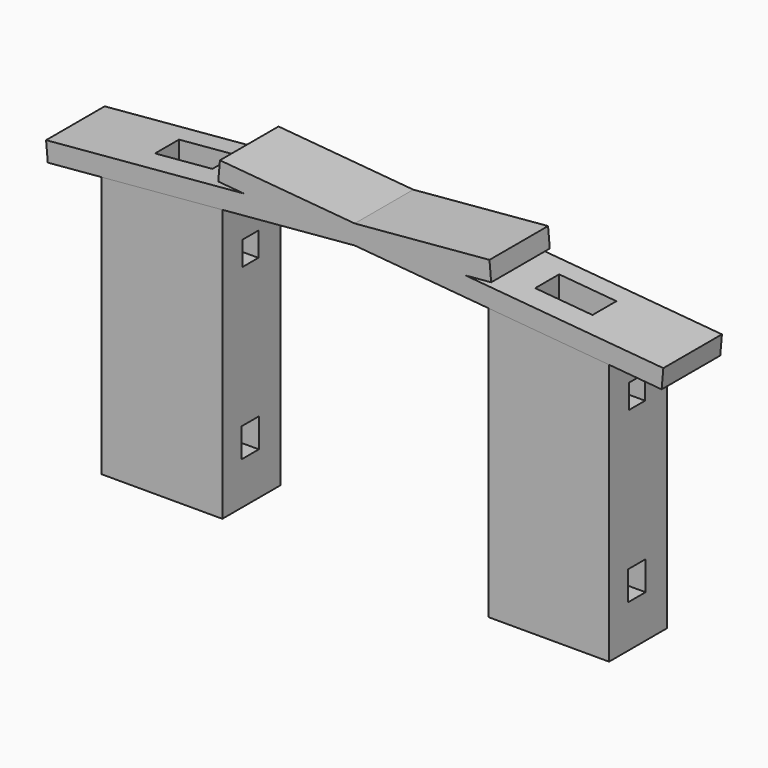
from build123d import *

# Parameters (mm, degrees)
F0_W      = 6.35
F0_H      = 6.35
F1_DEPTH  = 76.2
F3_W      = 78.9158530533
F3_H      = 6.5545327961
F4_DEPTH  = 5.08
F5_DEPTH  = 38.1
F7_DEPTH  = 25.4
F8_DEPTH  = 25.4
F9_DEPTH  = 12.7
F10_DEPTH = 12.7
F11_W     = 15.0663554668
F11_H     = 7.8755952418
F12_DEPTH = 88.9
F13_W     = 5.7417834178
F13_H     = 7.6454
F14_DEPTH = 2540
F15_W     = 5.208699964
F15_H     = 6.3248500228
F16_DEPTH = 25400


# Not quite as in the source:
# - a feature names something its author has since deleted; it is built from what else it names


with BuildPart() as f1:
    # F0 (on Top) → F1 (new body)
    with BuildSketch(Plane.XY):
        with Locations((-38.1329911691, -3.175)):
            Rectangle(F0_W, F0_H)
    extrude(amount=F1_DEPTH)

    # F3 (on face) → F4 (join)
    with BuildSketch(Plane(origin=(-6.9297761713, 0, 79.2077040846), x_dir=(0.9961946981, 0, 0.0871557427), z_dir=(0.0871557427, 0, -0.9961946981))):
        with Locations((3.0671004206, 3.2772663981)):
            Rectangle(F3_W, F3_H)
    extrude(amount=F4_DEPTH)

    # F5 (add): a face of the model
    f5_faces = [f1.faces().sort_by_distance(p)[0] for p in [
        (-42.9607486108, -3.2772663981, 73.5057000729),
    ]]
    extrude(f5_faces, amount=F5_DEPTH)

    # F6: F1 across plane


with BuildPart() as f1_1:
    add(f1.part)
    add(f1.part.mirror(Plane.YZ))

    # F7 (add): a face of the model
    f7_faces = [f1_1.faces().sort_by_distance(p)[0] for p in [
        (-41.3079911691, -3.175, 35.5502976126),
    ]]
    extrude(f7_faces, amount=F7_DEPTH)

    # F8 (add): a face of the model
    f8_faces = [f1_1.faces().sort_by_distance(p)[0] for p in [
        (41.3079911691, -3.175, 35.5502976126),
    ]]
    extrude(f8_faces, amount=F8_DEPTH)

    # F9 (add): a face of the model
    f9_faces = [f1_1.faces().sort_by_distance(p)[0] for p in [
        (0, -6.5545327961, 75.0015171841),
    ]]
    extrude(f9_faces, amount=F9_DEPTH)

    # F10 (add): faces of the model
    f10_faces = [f1_1.faces().sort_by_distance(p)[0] for p in [
        (-50.72839761, -6.35, 35.1382082279),
        (50.72839761, -6.35, 35.1382082279),
    ]]
    extrude(f10_faces, amount=F10_DEPTH)

    # F11 (on face) → F12 (cut)
    with BuildSketch(Plane(origin=(0, 0, 0), x_dir=(1, 0, 0), z_dir=(0, 0, -1))):
        with Locations((-49.9696880579, 9.0547855943)):
            Rectangle(F11_W, F11_H)
        with Locations((49.9696880579, 9.0547855943)):
            Rectangle(F11_W, F11_H)
    extrude(amount=-F12_DEPTH, mode=Mode.SUBTRACT)

    # F13 (on face) → F14 (cut)
    with BuildSketch(Plane(origin=(-66.7079911691, 0, 0), x_dir=(0, -1, 0), z_dir=(-1, 0, 0))):
        with Locations((9.922655765, 15.0297441246)):
            Rectangle(F13_W, F13_H)
    extrude(amount=-F14_DEPTH, mode=Mode.SUBTRACT)

    # F15 (on face) → F16 (cut)
    with BuildSketch(Plane(origin=(-66.7079911691, 0, 0), x_dir=(0, -1, 0), z_dir=(-1, 0, 0))):
        with Locations((9.8132924177, 58.757327497)):
            Rectangle(F15_W, F15_H)
    extrude(amount=-F16_DEPTH, mode=Mode.SUBTRACT)


solid = f1_1.part
